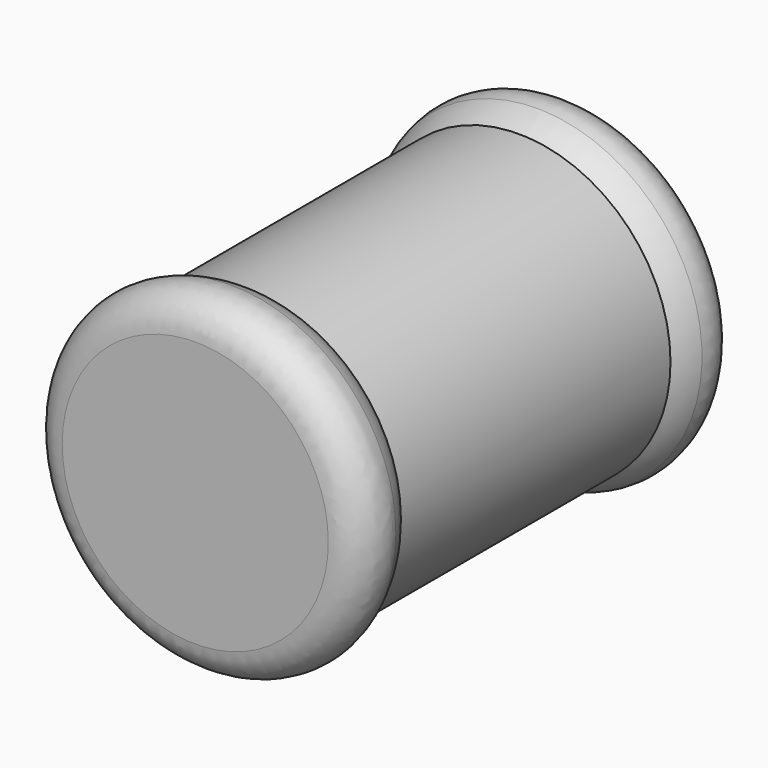
from build123d import *

# Parameters (mm, degrees)
F0_R     = 2.25
F1_DEPTH = 5
F2_R     = 2.5
F2_R_2   = 2.25
F3_DEPTH = 1
F5_R     = 0.5
F6_R     = 2.5
F6_R_2   = 2.25
F7_DEPTH = 1
F9_R     = 0.5


# Not quite as in the source:
# - a fillet or chamfer that OpenCascade refuses, or shapes differently, is made with other operations: its cross-section is extruded or revolved along the edge and cut away or added


with BuildPart() as f1:
    # F0 (on Front) → F1 (new body)
    with BuildSketch(Plane.XZ):
        Circle(F0_R)
    extrude(amount=F1_DEPTH)

    # F2 (on face) → F3 (join)
    with BuildSketch(Plane.XZ.offset(5)):
        Circle(F2_R)
        Circle(F2_R_2, mode=Mode.SUBTRACT)
        Circle(F2_R_2)
    extrude(amount=F3_DEPTH)

    # F4: fillet of radius 1 on 1 edges, made by hand

    # F4_s1 → F4_t2 (revolve, cut)
    with BuildSketch(Plane.XY):
        with BuildLine():
            ThreePointArc((2.5, -5.6614378278), (2.4354143467, -5.3078844372), (2.25, -5))
            Line((2.25, -5), (2.5, -5))
            Line((2.5, -5), (2.5, -5.6614378278))
        make_face()
    revolve(axis=Axis((0, -5, 0), (0, -1, 0)), mode=Mode.SUBTRACT)

    # F5
    f5_edges = [f1.edges().sort_by_distance(p)[0] for p in [
        (-2.5, -6, 0),
    ]]
    fillet(f5_edges, radius=F5_R)

    # F6 (on face) → F7 (join)
    with BuildSketch(Plane(origin=(0, 0, 0), x_dir=(-1, 0, 0), z_dir=(0, 1, 0))):
        Circle(F6_R)
        Circle(F6_R_2, mode=Mode.SUBTRACT)
        Circle(F6_R_2)
    extrude(amount=F7_DEPTH)

    # F8: fillet of radius 1 on 1 edges, made by hand

    # F8_s1 → F8_t2 (revolve, cut)
    with BuildSketch(Plane.XY):
        with BuildLine():
            ThreePointArc((-2.5, 0.6614378278), (-2.4354143467, 0.3078844372), (-2.25, 0))
            Line((-2.25, 0), (-2.5, 0))
            Line((-2.5, 0), (-2.5, 0.6614378278))
        make_face()
    revolve(axis=Axis((0, 0, 0), (0, 1, 0)), mode=Mode.SUBTRACT)

    # F9
    f9_edges = [f1.edges().sort_by_distance(p)[0] for p in [
        (2.5, 1, 0),
    ]]
    fillet(f9_edges, radius=F9_R)


solid = f1.part
